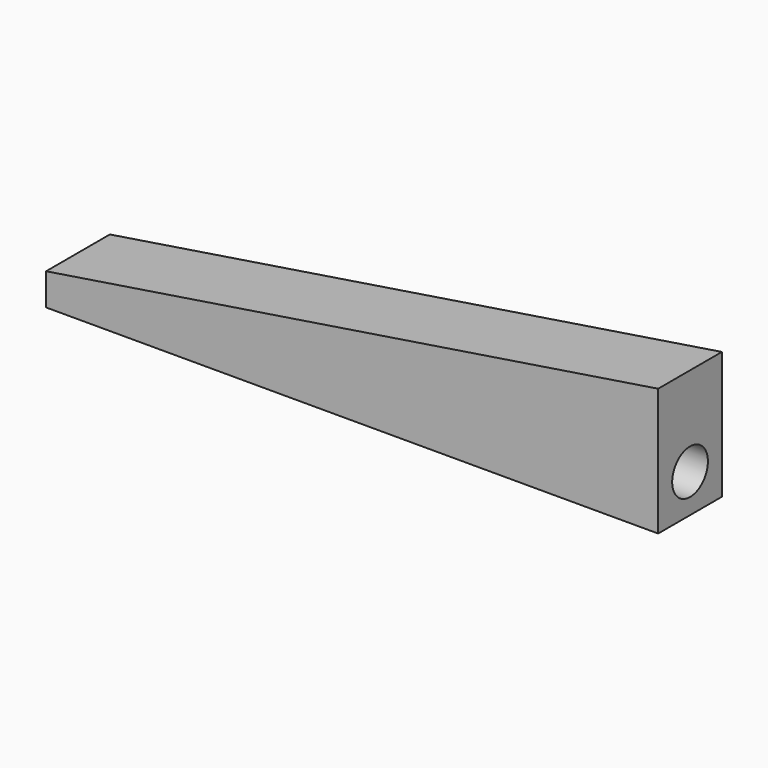
from build123d import *

# Parameters (mm, degrees)
F0_W     = 304.8
F0_H     = 63.5
F1_DEPTH = 39.6875
F2_SIZE2 = 304.79999
F2_SIZE  = 47.62499
F3_R     = 11.1125
F4_DEPTH = 50.8


# Not quite as in the source:
# - a fillet or chamfer is up to 0.001 mm smaller than in the source, because OpenCascade refuses the exact size
# - a length typed as a fraction of an inch, garbled in the dataset ("3 / 203.2 mm" for 3/8 in), is restored


with BuildPart() as f1:
    # F0 (on Front) → F1 (new body)
    with BuildSketch(Plane.XZ):
        with Locations((152.4, 31.75)):
            Rectangle(F0_W, F0_H)
    extrude(amount=F1_DEPTH)

    # F2 (size 47.625 and 304.8 in the source; OpenCascade refuses exactly that, so slightly less here)
    f2_edges = [f1.edges().sort_by_distance(p)[0] for p in [
        (0, -19.84375, 63.5),
    ]]
    f2_side = f1.faces().sort_by_distance((0, -19.84375, 31.75))[0]
    chamfer(f2_edges, length=F2_SIZE, length2=F2_SIZE2, reference=f2_side)

    # F3 (on face) → F4 (cut)
    with BuildSketch(Plane.YZ.offset(304.8)):
        with Locations((-19.84375, 19.05)):
            Circle(F3_R)
    extrude(amount=-F4_DEPTH, mode=Mode.SUBTRACT)


solid = f1.part
